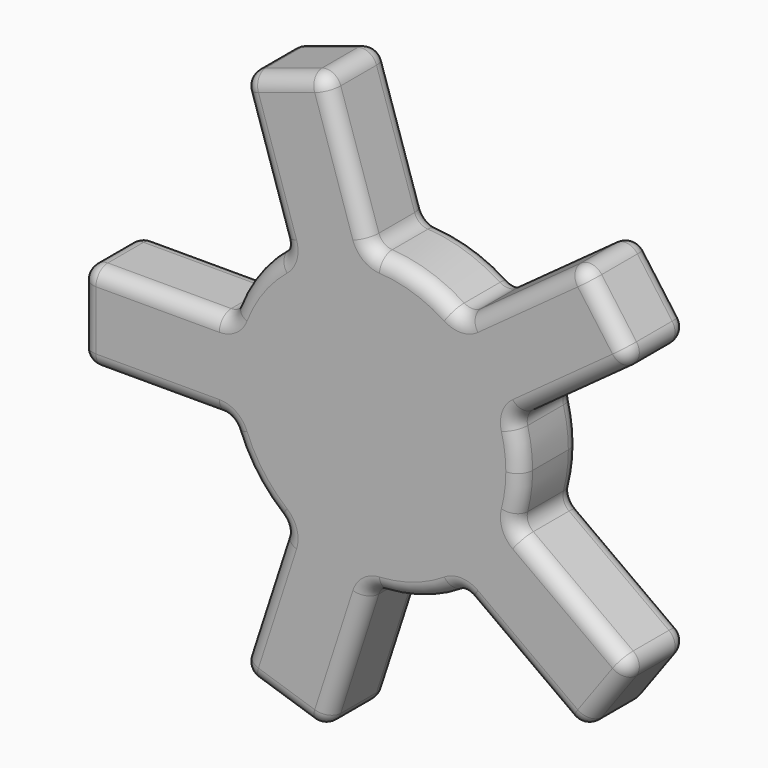
from build123d import *

# Parameters (mm, degrees)
F1_DEPTH = 12.7
F2_R     = 2.54
F3_R     = 2.54
F4_R     = 12.7
F5_DEPTH = 19.05
F6_SIZE  = 7.62


with BuildPart() as f1:
    # F0 (on Front) → F1 (new body)
    with BuildSketch(Plane.XZ):
        with BuildLine():
            ThreePointArc((24.2404523262, -7.5868617372), (25.1084397075, -3.8374803526), (25.4, 0))
            ThreePointArc((25.4, 0), (25.1084397075, 3.8374803526), (24.2404523262, 7.5868617372))
            Line((24.2404523262, 7.5868617372), (24.2404523262, -7.5868617372))
        make_face()
        with BuildLine():
            Line((23.3499594674, 7.5868617372), (24.2404523262, 7.5868617372))
            ThreePointArc((24.2404523262, 7.5868617372), (24.1568355139, 7.8490316571), (24.0703833236, 8.1102803069))
            Line((24.0703833236, 8.1102803069), (23.3499594674, 7.5868617372))
        make_face()
        Polygon((24.2404523262, -7.5868617372), (24.2404523262, 7.5868617372), (23.3499594674, 7.5868617372), (12.9075401392, 0), (23.3499594674, -7.5868617372), align=None)
        with BuildLine():
            ThreePointArc((24.0703833236, -8.1102803069), (24.1568355139, -7.8490316571), (24.2404523262, -7.5868617372))
            Line((24.2404523262, -7.5868617372), (23.3499594674, -7.5868617372))
            Line((23.3499594674, -7.5868617372), (24.0703833236, -8.1102803069))
        make_face()
        with BuildLine():
            Line((23.3499594674, 7.5868617372), (24.0703833236, 8.1102803069))
            ThreePointArc((24.0703833236, 8.1102803069), (20.5490316571, 14.9297454082), (15.151492443, 20.3860804656))
            Line((15.151492443, 20.3860804656), (14.4310685868, 19.8626618959))
            Line((14.4310685868, 19.8626618959), (10.4424193282, 7.5868617372))
            Line((10.4424193282, 7.5868617372), (23.3499594674, 7.5868617372))
        make_face()
        with BuildLine():
            ThreePointArc((15.151492443, 20.3860804656), (20.5490316571, 14.9297454082), (24.0703833236, 8.1102803069))
            Line((24.0703833236, 8.1102803069), (44.6194149807, 23.0400257151))
            Line((44.6194149807, 23.0400257151), (35.7005241001, 35.3158258738))
            Line((35.7005241001, 35.3158258738), (15.151492443, 20.3860804656))
        make_face()
        with BuildLine():
            Line((44.6194149807, -23.0400257151), (24.0703833236, -8.1102803069))
            ThreePointArc((24.0703833236, -8.1102803069), (20.5490316571, -14.9297454082), (15.151492443, -20.3860804656))
            Line((15.151492443, -20.3860804656), (35.7005241001, -35.3158258738))
            Line((35.7005241001, -35.3158258738), (44.6194149807, -23.0400257151))
        make_face()
        with BuildLine():
            ThreePointArc((15.151492443, -20.3860804656), (20.5490316571, -14.9297454082), (24.0703833236, -8.1102803069))
            Line((24.0703833236, -8.1102803069), (23.3499594674, -7.5868617372))
            Line((23.3499594674, -7.5868617372), (10.4424193282, -7.5868617372))
            Line((10.4424193282, -7.5868617372), (14.4310685868, -19.8626618959))
            Line((14.4310685868, -19.8626618959), (15.151492443, -20.3860804656))
        make_face()
        with BuildLine():
            Line((14.4310685868, 19.8626618959), (15.151492443, 20.3860804656))
            ThreePointArc((15.151492443, 20.3860804656), (14.9297454082, 20.5490316571), (14.7062460135, 20.7095709321))
            Line((14.7062460135, 20.7095709321), (14.4310685868, 19.8626618959))
        make_face()
        with BuildLine():
            ThreePointArc((14.7062460135, -20.7095709321), (14.9297454082, -20.5490316571), (15.151492443, -20.3860804656))
            Line((15.151492443, -20.3860804656), (14.4310685868, -19.8626618959))
            Line((14.4310685868, -19.8626618959), (14.7062460135, -20.7095709321))
        make_face()
        with BuildLine():
            Line((0.2751774268, 25.3985093536), (14.7062460135, 20.7095709321))
            ThreePointArc((14.7062460135, 20.7095709321), (7.8490316571, 24.1568355139), (0.2751774268, 25.3985093536))
        make_face()
        Polygon((14.4310685868, 19.8626618959), (14.7062460135, 20.7095709321), (0.2751774268, 25.3985093536), (0, 24.5516003174), (3.9886492586, 12.2758001587), align=None)
        Polygon((0.2751774268, -25.3985093536), (14.7062460135, -20.7095709321), (14.4310685868, -19.8626618959), (3.9886492586, -12.2758001587), (0, -24.5516003174), align=None)
        with BuildLine():
            ThreePointArc((0.2751774268, -25.3985093536), (7.8490316571, -24.1568355139), (14.7062460135, -20.7095709321))
            Line((14.7062460135, -20.7095709321), (0.2751774268, -25.3985093536))
        make_face()
        with BuildLine():
            Line((0, 24.5516003174), (0.2751774268, 25.3985093536))
            ThreePointArc((0.2751774268, 25.3985093536), (0, 25.4), (-0.2751774268, 25.3985093536))
            Line((-0.2751774268, 25.3985093536), (0, 24.5516003174))
        make_face()
        with BuildLine():
            ThreePointArc((-0.2751774268, -25.3985093536), (0, -25.4), (0.2751774268, -25.3985093536))
            Line((0.2751774268, -25.3985093536), (0, -24.5516003174))
            Line((0, -24.5516003174), (-0.2751774268, -25.3985093536))
        make_face()
        with BuildLine():
            Line((0, 24.5516003174), (-0.2751774268, 25.3985093536))
            ThreePointArc((-0.2751774268, 25.3985093536), (-7.8490316571, 24.1568355139), (-14.7062460135, 20.7095709321))
            Line((-14.7062460135, 20.7095709321), (-14.4310685868, 19.8626618959))
            Line((-14.4310685868, 19.8626618959), (-3.9886492586, 12.2758001587))
            Line((-3.9886492586, 12.2758001587), (0, 24.5516003174))
        make_face()
        with BuildLine():
            ThreePointArc((-14.7062460135, 20.7095709321), (-7.8490316571, 24.1568355139), (-0.2751774268, 25.3985093536))
            Line((-0.2751774268, 25.3985093536), (-8.1242090839, 49.5553448675))
            Line((-8.1242090839, 49.5553448675), (-22.5552776706, 44.8664064459))
            Line((-22.5552776706, 44.8664064459), (-14.7062460135, 20.7095709321))
        make_face()
        with BuildLine():
            Line((-8.1242090839, -49.5553448675), (-0.2751774268, -25.3985093536))
            ThreePointArc((-0.2751774268, -25.3985093536), (-7.8490316571, -24.1568355139), (-14.7062460135, -20.7095709321))
            Line((-14.7062460135, -20.7095709321), (-22.5552776706, -44.8664064459))
            Line((-22.5552776706, -44.8664064459), (-8.1242090839, -49.5553448675))
        make_face()
        with BuildLine():
            ThreePointArc((-14.7062460135, -20.7095709321), (-7.8490316571, -24.1568355139), (-0.2751774268, -25.3985093536))
            Line((-0.2751774268, -25.3985093536), (0, -24.5516003174))
            Line((0, -24.5516003174), (-3.9886492586, -12.2758001587))
            Line((-3.9886492586, -12.2758001587), (-14.4310685868, -19.8626618959))
            Line((-14.4310685868, -19.8626618959), (-14.7062460135, -20.7095709321))
        make_face()
        with BuildLine():
            Line((-14.4310685868, 19.8626618959), (-14.7062460135, 20.7095709321))
            ThreePointArc((-14.7062460135, 20.7095709321), (-14.9297454082, 20.5490316571), (-15.151492443, 20.3860804656))
            Line((-15.151492443, 20.3860804656), (-14.4310685868, 19.8626618959))
        make_face()
        with BuildLine():
            ThreePointArc((-15.151492443, -20.3860804656), (-14.9297454082, -20.5490316571), (-14.7062460135, -20.7095709321))
            Line((-14.7062460135, -20.7095709321), (-14.4310685868, -19.8626618959))
            Line((-14.4310685868, -19.8626618959), (-15.151492443, -20.3860804656))
        make_face()
        with BuildLine():
            Line((-24.0703833236, 8.1102803069), (-15.151492443, 20.3860804656))
            ThreePointArc((-15.151492443, 20.3860804656), (-20.5490316571, 14.9297454082), (-24.0703833236, 8.1102803069))
        make_face()
        Polygon((-14.4310685868, 19.8626618959), (-15.151492443, 20.3860804656), (-24.0703833236, 8.1102803069), (-23.3499594674, 7.5868617372), (-10.4424193282, 7.5868617372), align=None)
        Polygon((-24.0703833236, -8.1102803069), (-15.151492443, -20.3860804656), (-14.4310685868, -19.8626618959), (-10.4424193282, -7.5868617372), (-23.3499594674, -7.5868617372), align=None)
        with BuildLine():
            ThreePointArc((-24.0703833236, -8.1102803069), (-20.5490316571, -14.9297454082), (-15.151492443, -20.3860804656))
            Line((-15.151492443, -20.3860804656), (-24.0703833236, -8.1102803069))
        make_face()
        with BuildLine():
            Line((-23.3499594674, 7.5868617372), (-24.0703833236, 8.1102803069))
            ThreePointArc((-24.0703833236, 8.1102803069), (-24.1568355139, 7.8490316571), (-24.2404523262, 7.5868617372))
            Line((-24.2404523262, 7.5868617372), (-23.3499594674, 7.5868617372))
        make_face()
        with BuildLine():
            Line((-12.9075401392, 0), (-23.3499594674, 7.5868617372))
            Line((-23.3499594674, 7.5868617372), (-24.2404523262, 7.5868617372))
            ThreePointArc((-24.2404523262, 7.5868617372), (-25.1084397075, 3.8374803526), (-25.4, 0))
            Line((-25.4, 0), (-12.9075401392, 0))
        make_face()
        with BuildLine():
            Line((-23.3499594674, -7.5868617372), (-12.9075401392, 0))
            Line((-12.9075401392, 0), (-25.4, 0))
            ThreePointArc((-25.4, 0), (-25.1084397075, -3.8374803526), (-24.2404523262, -7.5868617372))
            Line((-24.2404523262, -7.5868617372), (-23.3499594674, -7.5868617372))
        make_face()
        with BuildLine():
            ThreePointArc((-24.2404523262, -7.5868617372), (-24.1568355139, -7.8490316571), (-24.0703833236, -8.1102803069))
            Line((-24.0703833236, -8.1102803069), (-23.3499594674, -7.5868617372))
            Line((-23.3499594674, -7.5868617372), (-24.2404523262, -7.5868617372))
        make_face()
        with BuildLine():
            ThreePointArc((-25.4, 0), (-25.1084397075, 3.8374803526), (-24.2404523262, 7.5868617372))
            Line((-24.2404523262, 7.5868617372), (-49.6404523262, 7.5868617372))
            Line((-49.6404523262, 7.5868617372), (-49.6404523262, -7.5868617372))
            Line((-49.6404523262, -7.5868617372), (-24.2404523262, -7.5868617372))
            ThreePointArc((-24.2404523262, -7.5868617372), (-25.1084397075, -3.8374803526), (-25.4, 0))
        make_face()
        Polygon((6.4537700696, 4.6889384215), (2.465120811, 7.5868617372), (-2.465120811, 7.5868617372), (-6.4537700696, 4.6889384215), (-7.9772985172, 0), (-6.4537700696, -4.6889384215), (-2.465120811, -7.5868617372), (2.465120811, -7.5868617372), (6.4537700696, -4.6889384215), (7.9772985172, 0), align=None)
        Polygon((0, 9.3778768431), (3.9886492586, 12.2758001587), (0, 24.5516003174), (-3.9886492586, 12.2758001587), align=None)
        Polygon((5.5121777062, 7.5868617372), (10.4424193282, 7.5868617372), (14.4310685868, 19.8626618959), (3.9886492586, 12.2758001587), align=None)
        Polygon((12.9075401392, 0), (23.3499594674, 7.5868617372), (10.4424193282, 7.5868617372), (8.9188908806, 2.8979233157), align=None)
        Polygon((10.4424193282, -7.5868617372), (23.3499594674, -7.5868617372), (12.9075401392, 0), (8.9188908806, -2.8979233157), align=None)
        Polygon((-14.4310685868, -19.8626618959), (-3.9886492586, -12.2758001587), (-5.5121777062, -7.5868617372), (-10.4424193282, -7.5868617372), align=None)
        Polygon((14.4310685868, -19.8626618959), (10.4424193282, -7.5868617372), (5.5121777062, -7.5868617372), (3.9886492586, -12.2758001587), align=None)
        Polygon((3.9886492586, -12.2758001587), (5.5121777062, -7.5868617372), (2.465120811, -7.5868617372), (0, -9.3778768431), align=None)
        Polygon((-3.9886492586, -12.2758001587), (0, -9.3778768431), (-2.465120811, -7.5868617372), (-5.5121777062, -7.5868617372), align=None)
        Polygon((-8.9188908806, -2.8979233157), (-7.9772985172, 0), (-12.9075401392, 0), align=None)
        Polygon((-8.9188908806, 2.8979233157), (-10.4424193282, 7.5868617372), (-23.3499594674, 7.5868617372), (-12.9075401392, 0), align=None)
        Polygon((-5.5121777062, 7.5868617372), (-3.9886492586, 12.2758001587), (-14.4310685868, 19.8626618959), (-10.4424193282, 7.5868617372), align=None)
        Polygon((0, -24.5516003174), (3.9886492586, -12.2758001587), (0, -9.3778768431), (-3.9886492586, -12.2758001587), align=None)
        Polygon((-23.3499594674, -7.5868617372), (-10.4424193282, -7.5868617372), (-8.9188908806, -2.8979233157), (-12.9075401392, 0), align=None)
        Polygon((-10.4424193282, -7.5868617372), (-5.5121777062, -7.5868617372), (-6.4537700696, -4.6889384215), (-8.9188908806, -2.8979233157), align=None)
        Polygon((-8.9188908806, -2.8979233157), (-6.4537700696, -4.6889384215), (-7.9772985172, 0), align=None)
        Polygon((-12.9075401392, 0), (-7.9772985172, 0), (-8.9188908806, 2.8979233157), align=None)
        Polygon((-6.4537700696, 4.6889384215), (-5.5121777062, 7.5868617372), (-10.4424193282, 7.5868617372), (-8.9188908806, 2.8979233157), align=None)
        Polygon((-2.465120811, 7.5868617372), (0, 9.3778768431), (-3.9886492586, 12.2758001587), (-5.5121777062, 7.5868617372), align=None)
        Polygon((2.465120811, 7.5868617372), (5.5121777062, 7.5868617372), (3.9886492586, 12.2758001587), (0, 9.3778768431), align=None)
        Polygon((6.4537700696, 4.6889384215), (5.5121777062, 7.5868617372), (2.465120811, 7.5868617372), align=None)
        Polygon((8.9188908806, -2.8979233157), (12.9075401392, 0), (8.9188908806, 2.8979233157), (7.9772985172, 0), align=None)
        Polygon((7.9772985172, 0), (8.9188908806, 2.8979233157), (6.4537700696, 4.6889384215), align=None)
        Polygon((6.4537700696, -4.6889384215), (8.9188908806, -2.8979233157), (7.9772985172, 0), align=None)
        Polygon((0, -9.3778768431), (2.465120811, -7.5868617372), (-2.465120811, -7.5868617372), align=None)
        Polygon((-5.5121777062, -7.5868617372), (-2.465120811, -7.5868617372), (-6.4537700696, -4.6889384215), align=None)
        Polygon((-7.9772985172, 0), (-6.4537700696, 4.6889384215), (-8.9188908806, 2.8979233157), align=None)
        Polygon((-6.4537700696, 4.6889384215), (-2.465120811, 7.5868617372), (-5.5121777062, 7.5868617372), align=None)
        Polygon((-2.465120811, 7.5868617372), (2.465120811, 7.5868617372), (0, 9.3778768431), align=None)
        Polygon((8.9188908806, 2.8979233157), (10.4424193282, 7.5868617372), (5.5121777062, 7.5868617372), (6.4537700696, 4.6889384215), align=None)
        Polygon((5.5121777062, -7.5868617372), (10.4424193282, -7.5868617372), (8.9188908806, -2.8979233157), (6.4537700696, -4.6889384215), align=None)
        Polygon((2.465120811, -7.5868617372), (5.5121777062, -7.5868617372), (6.4537700696, -4.6889384215), align=None)
    extrude(amount=F1_DEPTH)

    # F2
    f2_edges = [f1.edges().sort_by_distance(p)[0] for p in [
        (44.619415, -6.35, 23.040026),
        (44.619415, -6.35, -23.040026),
        (35.700524, -6.35, -35.315826),
        (-8.124209, -6.35, -49.555345),
        (-22.555278, -6.35, -44.866406),
        (-49.640452, -6.35, -7.586862),
        (-49.640452, -6.35, 7.586862),
        (35.700524, -6.35, 35.315826),
        (-8.124209, -6.35, 49.555345),
        (-22.555278, -6.35, 44.866406),
    ]]
    fillet(f2_edges, radius=F2_R)

    # F3
    f3_edges = [f1.edges().sort_by_distance(p)[0] for p in [
        (7.849032, 0, 24.156836),
        (-20.549032, 0, 14.929745),
        (7.849032, -12.7, 24.156836),
        (-20.549032, -12.7, 14.929745),
        (25.4, -12.7, 0),
        (25.4, 0, 0),
        (24.070383, -6.35, -8.11028),
        (24.070383, -6.35, 8.11028),
        (-14.706246, -6.35, 20.709571),
        (-24.240452, -6.35, 7.586862),
        (15.151492, -6.35, 20.38608),
        (-0.275177, -6.35, 25.398509),
        (-24.240452, -6.35, -7.586862),
        (-14.706246, -6.35, -20.709571),
        (-20.549032, 0, -14.929745),
        (-20.549032, -12.7, -14.929745),
        (33.317448, 0, 14.828666),
        (33.317448, -12.7, 14.828666),
        (43.580266, 0, 23.204611),
        (40.15997, 0, 29.177926),
        (33.317448, 0, -14.828666),
        (35.535939, 0, 34.276677),
        (43.580266, 0, -23.204611),
        (24.398557, 0, 27.104466),
        (40.15997, 0, -29.177926),
        (35.535939, 0, -34.276677),
        (-3.807242, 0, 36.269085),
        (24.398557, 0, -27.104466),
        (-8.601854, 0, 48.617915),
        (7.849032, 0, -24.156836),
        (-15.339743, 0, 47.210876),
        (-3.807242, 0, -36.269085),
        (-21.617848, 0, 44.388762),
        (-8.601854, 0, -48.617915),
        (-18.23831, 0, 31.580147),
        (-15.339743, 0, -47.210876),
        (-21.617848, 0, -44.388762),
        (-35.670452, 0, 7.586862),
        (-18.23831, 0, -31.580147),
        (-48.896504, 0, 6.842913),
        (-49.640452, 0, 0),
        (-35.670452, 0, -7.586862),
        (-48.896504, 0, -6.842913),
        (43.580266, -12.7, 23.204611),
        (40.15997, -12.7, 29.177926),
        (33.317448, -12.7, -14.828666),
        (35.535939, -12.7, 34.276677),
        (43.580266, -12.7, -23.204611),
        (24.398557, -12.7, 27.104466),
        (40.15997, -12.7, -29.177926),
        (35.535939, -12.7, -34.276677),
        (-3.807242, -12.7, 36.269085),
        (24.398557, -12.7, -27.104466),
        (-8.601854, -12.7, 48.617915),
        (7.849032, -12.7, -24.156836),
        (-15.339743, -12.7, 47.210876),
        (-3.807242, -12.7, -36.269085),
        (-21.617848, -12.7, 44.388762),
        (-8.601854, -12.7, -48.617915),
        (-18.23831, -12.7, 31.580147),
        (-15.339743, -12.7, -47.210876),
        (-21.617848, -12.7, -44.388762),
        (-35.670452, -12.7, 7.586862),
        (-18.23831, -12.7, -31.580147),
        (-48.896504, -12.7, 6.842913),
        (-49.640452, -12.7, 0),
        (-35.670452, -12.7, -7.586862),
        (-48.896504, -12.7, -6.842913),
        (15.151492, -6.35, -20.38608),
        (-0.275177, -6.35, -25.398509),
    ]]
    fillet(f3_edges, radius=F3_R)

    # F4 (on face) → F5 (join)
    with BuildSketch(Plane(origin=(0, 0, 0), x_dir=(-1, 0, 0), z_dir=(0, 1, 0))):
        Circle(F4_R)
    extrude(amount=F5_DEPTH)

    # F6
    f6_edges = [f1.edges().sort_by_distance(p)[0] for p in [
        (12.7, 19.05, 0),
    ]]
    chamfer(f6_edges, length=F6_SIZE)


solid = f1.part
